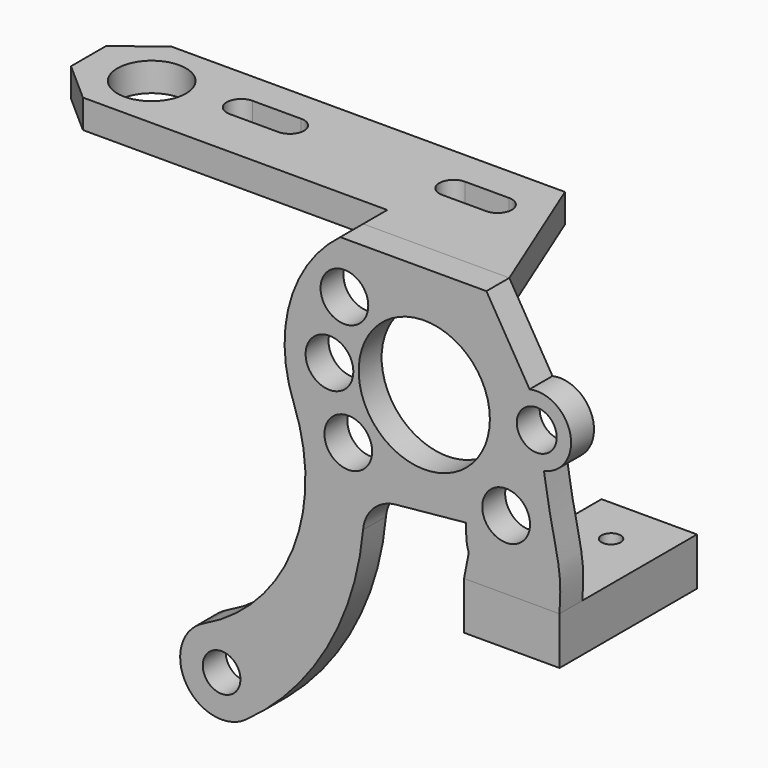
from build123d import *

# Parameters (mm, degrees)
F0_W     = 10
F0_H     = 18
F0_R     = 1.6
F0_R_2   = 1
F1_DEPTH = 5
F2_R     = 1.9699121269
F2_R_2   = 2.5
F2_R_3   = 6.869499788
F2_R_4   = 2.0896484604
F3_DEPTH = 3
F4_R     = 3.5880472774
F5_DEPTH = 3
F7_DEPTH = 3.1614936367


with BuildPart() as f1:
    # F0 (on Top) → F1 (new body)
    with BuildSketch(Plane.XY):
        with Locations((-8.3221568636, 1.0862629861)):
            Rectangle(F0_W, F0_H)
        with Locations((-8.3221568636, -1.9137370139)):
            Circle(F0_R, mode=Mode.SUBTRACT)
        with Locations((-8.3221568636, 5.0862629861)):
            Circle(F0_R_2, mode=Mode.SUBTRACT)
    extrude(amount=F1_DEPTH)


with BuildPart() as f3:
    # F2 (on face) → F3 (new body)
    with BuildSketch(Plane.XZ.offset(7.9137370139)):
        with BuildLine():
            Line((-13.3221568636, 5), (-3.3221568636, 5))
            add(Edge.make_bspline(
                [(-3.3221568636, 5), (-3.2552653311, 6.0908019939), (-3.0746854072, 9.342919926), (-4.269755775, 12.9369020162), (-4.9549108371, 17.6448374987)],
                knots=[0, 0, 0, 0, 0.3878947266, 1, 1, 1, 1], degree=3))
            ThreePointArc((-4.9549108371, 17.6448374987), (-2.1886315475, 21.9156040845), (-6.4593981333, 24.6818833741))
            Line((-6.4593981333, 24.6818833741), (-10.9792040735, 32.2593962774))
            Line((-10.9792040735, 32.2593962774), (-26.2877818286, 32.2593962774))
            ThreePointArc((-26.2877818286, 32.2593962774), (-31.547377506, 24.6142485357), (-31.1504669753, 15.3431055256))
            ThreePointArc((-31.1504669753, 15.3431055256), (-31.2702316577, 1.826680677), (-40.5582249678, -7.9937706638))
            ThreePointArc((-40.5582249678, -7.9937706638), (-42.4590174037, -14.1180551679), (-36.1872349298, -15.4539508117))
            ThreePointArc((-36.1872349298, -15.4539508117), (-27.6944192034, -6.0499089443), (-23.8997744182, 6.0399460324))
            ThreePointArc((-23.8997744182, 6.0399460324), (-22.8122929978, 8.3806310483), (-20.4814388049, 9.4890266975))
            Line((-20.4814388049, 9.4890266975), (-13.098238966, 10.2140815927))
            add(Edge.make_bspline(
                [(-13.3221568636, 5), (-12.3911872602, 9.2965995769), (-13.1695237687, 6.2813326191), (-13.098238966, 10.2140815927)],
                knots=[0, 0, 0, 0, 5.2188874371, 5.2188874371, 5.2188874371, 5.2188874371], degree=3))
        make_face()
        with Locations((-38.7134026542, -11.9234640947)):
            Circle(F2_R, mode=Mode.SUBTRACT)
        with Locations((-25.4434074495, 13.5795854718)):
            Circle(F2_R_2, mode=Mode.SUBTRACT)
        with Locations((-27.4161801418, 20.3022349277)):
            Circle(F2_R_2, mode=Mode.SUBTRACT)
        with Locations((-25.8515487019, 26.8880009391)):
            Circle(F2_R_2, mode=Mode.SUBTRACT)
        with Locations((-8.913740901, 12.2281657972)):
            Circle(F2_R_2, mode=Mode.SUBTRACT)
        with Locations((-17.4858285757, 20.5721753575)):
            Circle(F2_R_3, mode=Mode.SUBTRACT)
        with Locations((-5.7071544852, 21.1633604364)):
            Circle(F2_R_4, mode=Mode.SUBTRACT)
    extrude(amount=-F3_DEPTH)


with BuildPart() as f5:
    # F4 (on face) → F5 (new body)
    with BuildSketch(Plane.XY.offset(32.2593962774)):
        Polygon((-26.2877818286, -4.9137370139), (-10.9792040735, -4.9137370139), (-16.9395767152, 9.8199117929), (-58.1803768873, 9.8199117929), (-62.392167747, 6.5383897163), (-62.392167747, 1.9674218294), (-58.1693314016, -1.7522433773), (-26.2043997645, -1.7522433773), align=None)
        with Locations((-55.6143447757, 4.0625985712)):
            Circle(F4_R, mode=Mode.SUBTRACT)
        with BuildLine():
            Line((-46.9706878066, 6.4617942423), (-41.8741069734, 6.4617942423))
            ThreePointArc((-41.8741069734, 6.4617942423), (-40.3741069734, 4.9617942423), (-41.8741069734, 3.4617942423))
            Line((-41.8741069734, 3.4617942423), (-46.9706878066, 3.4617942423))
            ThreePointArc((-46.9706878066, 3.4617942423), (-48.4706878066, 4.9617942423), (-46.9706878066, 6.4617942423))
        make_face(mode=Mode.SUBTRACT)
        with BuildLine():
            Line((-24.4482420385, 6.1331547201), (-19.8469385505, 6.1331547201))
            ThreePointArc((-19.8469385505, 6.1331547201), (-18.3469385505, 4.6331547201), (-19.8469385505, 3.1331547201))
            Line((-19.8469385505, 3.1331547201), (-24.4482420385, 3.1331547201))
            ThreePointArc((-24.4482420385, 3.1331547201), (-25.9482420385, 4.6331547201), (-24.4482420385, 6.1331547201))
        make_face(mode=Mode.SUBTRACT)
    extrude(amount=-F5_DEPTH)

    # F6 (on face) → F7 (join, through all)
    with BuildSketch(Plane.XZ.offset(1.7522433773)):
        with BuildLine():
            Line((-26.2043997645, 32.2593962774), (-26.2877818286, 32.2593962774))
            ThreePointArc((-26.2877818286, 32.2593962774), (-27.8819639855, 30.8671198662), (-29.2585812948, 29.2593962774))
            Line((-29.2585812948, 29.2593962774), (-26.2043997645, 29.2593962774))
            Line((-26.2043997645, 29.2593962774), (-26.2043997645, 32.2593962774))
        make_face()
    extrude(amount=F7_DEPTH)


solid = Compound([f1.part, f3.part, f5.part])
